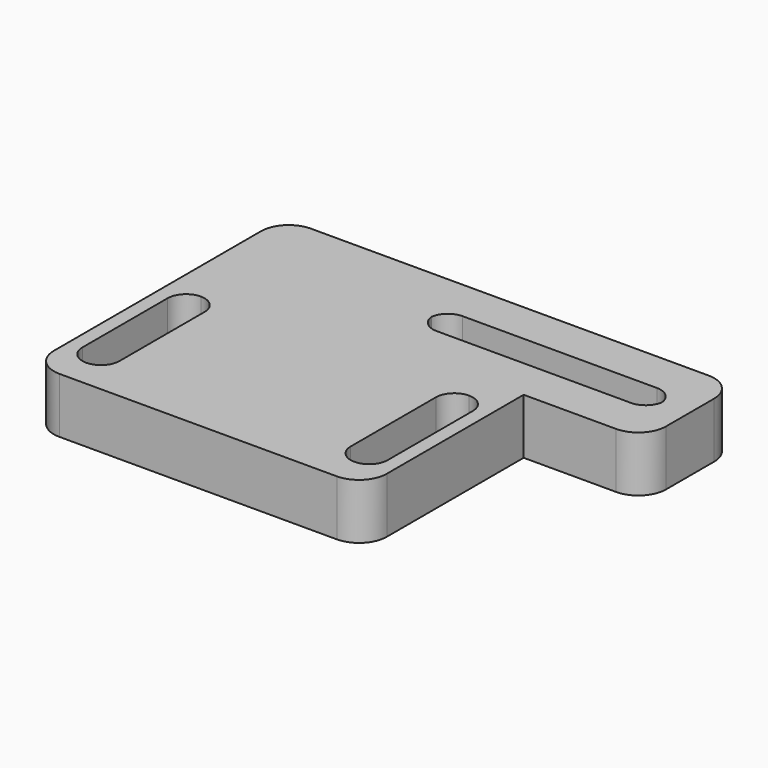
from build123d import *

# Parameters (mm, degrees)
F0_W        = 36
F0_H        = 21.5
F0_R        = 1.625
F0_W_2      = 4
F0_H_2      = 15.5
F0_W_3      = 25
F0_H_3      = 3.5
F1_DEPTH    = 6
F2_T1_DEPTH = 6
F3_R        = 3


# Not quite as in the source:
# - a fillet or chamfer that OpenCascade refuses, or shapes differently, is made with other operations: its cross-section is extruded or revolved along the edge and cut away or added


with BuildPart() as f1:
    # F0 (on Top) → F1 (new body)
    with BuildSketch(Plane.XY):
        Rectangle(F0_W, F0_H)
        with Locations((-4.0289468229, -6.686462095)):
            Circle(F0_R, mode=Mode.SUBTRACT)
        with Locations((4.0289468229, -6.686462095)):
            Circle(F0_R, mode=Mode.SUBTRACT)
        with Locations((-14.5, 0)):
            Rectangle(F0_W_2, F0_H_2, mode=Mode.SUBTRACT)
        with Locations((14.5, 0)):
            Rectangle(F0_W_2, F0_H_2, mode=Mode.SUBTRACT)
        Polygon((-18, 10.75), (18, 10.75), (31, 10.75), (31, 23.25), (-18, 23.25), align=None)
        with Locations((15.5, 17)):
            Rectangle(F0_W_3, F0_H_3, mode=Mode.SUBTRACT)
        with Locations((-4.0289468229, -6.686462095)):
            Circle(F0_R)
        with Locations((4.0289468229, -6.686462095)):
            Circle(F0_R)
    extrude(amount=F1_DEPTH)

    # F2: fillet of radius 2 on 12 edges, made by hand

    # F2_s2 → F2_t1 (join)
    with BuildSketch(Plane.XY):
        with BuildLine():
            ThreePointArc((3, 16.75), (3.5857864376, 18.1642135624), (5, 18.75))
            Line((5, 18.75), (3, 18.75))
            Line((3, 18.75), (3, 16.75))
        make_face()
        with BuildLine():
            ThreePointArc((26, 18.75), (27.4142135624, 18.1642135624), (28, 16.75))
            Line((28, 16.75), (28, 18.75))
            Line((28, 18.75), (26, 18.75))
        make_face()
        with BuildLine():
            ThreePointArc((28, 17.25), (27.4142135624, 15.8357864376), (26, 15.25))
            Line((26, 15.25), (28, 15.25))
            Line((28, 15.25), (28, 17.25))
        make_face()
        with BuildLine():
            ThreePointArc((3, 17.25), (3.5857864376, 15.8357864376), (5, 15.25))
            Line((5, 15.25), (3, 15.25))
            Line((3, 15.25), (3, 17.25))
        make_face()
        with BuildLine():
            ThreePointArc((-14.5, -7.75), (-15.9142135624, -7.1642135624), (-16.5, -5.75))
            Line((-16.5, -5.75), (-16.5, -7.75))
            Line((-16.5, -7.75), (-14.5, -7.75))
        make_face()
        with BuildLine():
            ThreePointArc((14.5, -7.75), (13.0857864376, -7.1642135624), (12.5, -5.75))
            Line((12.5, -5.75), (12.5, -7.75))
            Line((12.5, -7.75), (14.5, -7.75))
        make_face()
        with BuildLine():
            ThreePointArc((14.5, -7.75), (15.9142135624, -7.1642135624), (16.5, -5.75))
            Line((16.5, -5.75), (16.5, -7.75))
            Line((16.5, -7.75), (14.5, -7.75))
        make_face()
        with BuildLine():
            ThreePointArc((-12.5, -5.75), (-13.0857864376, -7.1642135624), (-14.5, -7.75))
            Line((-14.5, -7.75), (-12.5, -7.75))
            Line((-12.5, -7.75), (-12.5, -5.75))
        make_face()
        with BuildLine():
            ThreePointArc((-14.5, 7.75), (-13.0857864376, 7.1642135624), (-12.5, 5.75))
            Line((-12.5, 5.75), (-12.5, 7.75))
            Line((-12.5, 7.75), (-14.5, 7.75))
        make_face()
        with BuildLine():
            ThreePointArc((-14.5, 7.75), (-15.9142135624, 7.1642135624), (-16.5, 5.75))
            Line((-16.5, 5.75), (-16.5, 7.75))
            Line((-16.5, 7.75), (-14.5, 7.75))
        make_face()
        with BuildLine():
            ThreePointArc((12.5, 5.75), (13.0857864376, 7.1642135624), (14.5, 7.75))
            Line((14.5, 7.75), (12.5, 7.75))
            Line((12.5, 7.75), (12.5, 5.75))
        make_face()
        with BuildLine():
            ThreePointArc((14.5, 7.75), (15.9142135624, 7.1642135624), (16.5, 5.75))
            Line((16.5, 5.75), (16.5, 7.75))
            Line((16.5, 7.75), (14.5, 7.75))
        make_face()
    extrude(amount=F2_T1_DEPTH)

    # F3
    f3_edges = [f1.edges().sort_by_distance(p)[0] for p in [
        (31, 10.75, 3),
        (31, 23.25, 3),
        (-18, 23.25, 3),
        (-18, -10.75, 3),
        (18, -10.75, 3),
    ]]
    fillet(f3_edges, radius=F3_R)


solid = f1.part
